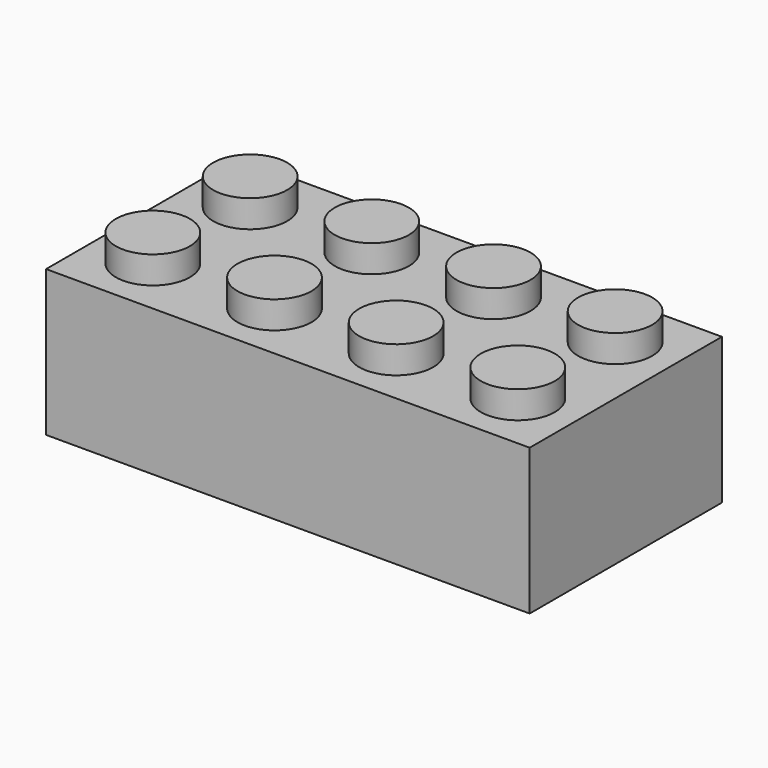
from build123d import *

# Parameters (mm, degrees)
F0_W        = 31.8
F0_H        = 15.8
F1_DEPTH    = 9.6
F2_R        = 2.435
F3_DEPTH    = 1.8
F4_T        = -1.24
F5_R        = 3.2
F6_DEPTH    = 8.36
F7_T        = 1.24
F7_T3_DEPTH = 10.84
F7_T5_DEPTH = 15.8
F7_T7_DEPTH = 31.8


# Not quite as in the source:
# - a shell that OpenCascade refuses in one call is made with other operations: the cavity is built on its own and cut out


with BuildPart() as f1:
    # F0 (on Top) → F1 (new body)
    with BuildSketch(Plane.XY):
        with Locations((15.9, 7.9)):
            Rectangle(F0_W, F0_H)
    extrude(amount=F1_DEPTH)

    # F2 (on face) → F3 (join)
    with BuildSketch(Plane.XY.offset(9.6)):
        with Locations((3.9, 11.9)):
            Circle(F2_R)
        with Locations((11.9, 11.9)):
            Circle(F2_R)
        with Locations((19.9, 11.9)):
            Circle(F2_R)
        with Locations((27.9, 11.9)):
            Circle(F2_R)
        with Locations((27.9, 3.9)):
            Circle(F2_R)
        with Locations((19.9, 3.9)):
            Circle(F2_R)
        with Locations((11.9, 3.9)):
            Circle(F2_R)
        with Locations((3.9, 3.9)):
            Circle(F2_R)
    extrude(amount=F3_DEPTH)

    # F4
    f4_openings = [f1.faces().sort_by_distance(p)[0] for p in [
        (15.9, 7.9, 0),
    ]]
    offset(amount=F4_T, openings=f4_openings, kind=Kind.INTERSECTION)

    # F5 (on face) → F6 (join)
    with BuildSketch(Plane(origin=(0, 0, 8.36), x_dir=(1, 0, 0), z_dir=(0, 0, -1))):
        with Locations((7.9, -7.9)):
            Circle(F5_R)
        with Locations((15.9, -7.9)):
            Circle(F5_R)
        with Locations((23.9, -7.9)):
            Circle(F5_R)
    extrude(amount=F6_DEPTH)

    # F7: shell of thickness 1.24, made by hand


with BuildPart() as f7_core1:
    # F7_t2: copy of F1
    add(f1.part)

    # the walls: a layer under each face that stays
    f7_faces = [f7_core1.faces().sort_by_distance(p)[0] for p in [
        (0, 7.9, 4.8),
        (15.9, 15.8, 4.8),
        (15.9, 0, 4.8),
        (2.2714285714, 1.1285714286, 0),
        (15.9, 7.9, 9.6),
        (31.8, 7.9, 4.8),
        (1.24, 7.9, 4.18),
        (15.9, 14.56, 4.18),
        (30.56, 7.9, 4.18),
        (15.9, 1.24, 4.18),
        (1.465, 3.9, 10.5),
        (9.465, 3.9, 10.5),
        (17.465, 3.9, 10.5),
        (25.465, 3.9, 10.5),
        (1.465, 11.9, 10.5),
        (9.465, 11.9, 10.5),
        (17.465, 11.9, 10.5),
        (25.465, 11.9, 10.5),
        (6.1266666667, 3.46, 8.36),
        (3.9, 3.9, 11.4),
        (11.9, 3.9, 11.4),
        (19.9, 3.9, 11.4),
        (27.9, 3.9, 11.4),
        (3.9, 11.9, 11.4),
        (11.9, 11.9, 11.4),
        (19.9, 11.9, 11.4),
        (27.9, 11.9, 11.4),
        (2.705, 3.9, 9.26),
        (10.705, 3.9, 9.26),
        (18.705, 3.9, 9.26),
        (26.705, 3.9, 9.26),
        (4.7, 7.9, 4.18),
        (2.705, 11.9, 9.26),
        (10.705, 11.9, 9.26),
        (12.7, 7.9, 4.18),
        (20.7, 7.9, 4.18),
        (18.705, 11.9, 9.26),
        (26.705, 11.9, 9.26),
        (3.9, 3.9, 10.16),
        (11.9, 3.9, 10.16),
        (19.9, 3.9, 10.16),
        (27.9, 3.9, 10.16),
        (3.9, 11.9, 10.16),
        (11.9, 11.9, 10.16),
        (19.9, 11.9, 10.16),
        (27.9, 11.9, 10.16),
    ]]
    thicken(f7_faces, amount=-F7_T, mode=Mode.SUBTRACT)

    # F7_s4 → F7_t3 (cut)
    with BuildSketch(Plane.XY.offset(-1.24)):
        Polygon((1.2524, 14.5476), (0, 14.56), (0, 15.8), (1.24, 15.8), align=None)
        Polygon((1.2524, 1.2524), (0, 1.24), (0, 0), (1.24, 0), align=None)
        Polygon((30.5476, 14.5476), (30.56, 15.8), (31.8, 15.8), (31.8, 14.56), align=None)
        Polygon((30.5476, 1.2524), (31.8, 1.24), (31.8, 0), (30.56, 0), align=None)
    extrude(amount=F7_T3_DEPTH, mode=Mode.SUBTRACT)

    # F7_s6 → F7_t5 (cut)
    with BuildSketch(Plane.XZ.offset(-15.8)):
        Polygon((1.2524, 8.3476), (0, 8.36), (0, 9.6), (1.24, 9.6), align=None)
        Polygon((30.5476, 8.3476), (31.8, 8.36), (31.8, 9.6), (30.56, 9.6), align=None)
    extrude(amount=F7_T5_DEPTH, mode=Mode.SUBTRACT)

    # F7_s8 → F7_t7 (cut)
    with BuildSketch(Plane.YZ):
        Polygon((14.5476, 8.3476), (15.8, 8.36), (15.8, 9.6), (14.56, 9.6), align=None)
        Polygon((1.2524, 8.3476), (0, 8.36), (0, 9.6), (1.24, 9.6), align=None)
    extrude(amount=F7_T7_DEPTH, mode=Mode.SUBTRACT)

    # F7_s9 → F7_t10 (revolve, cut)
    with BuildSketch(Plane.XZ.offset(-3.9)):
        Polygon((6.3474, 9.6124), (6.335, 8.36), (5.095, 8.36), (5.095, 9.6), align=None)
    revolve(axis=Axis((3.9, 3.9, 9.6), (0, 0, 1)), mode=Mode.SUBTRACT)

    # F7_s11 → F7_t12 (revolve, cut)
    with BuildSketch(Plane.XZ.offset(-3.9)):
        Polygon((14.3474, 9.6124), (14.335, 8.36), (13.095, 8.36), (13.095, 9.6), align=None)
    revolve(axis=Axis((11.9, 3.9, 9.6), (0, 0, 1)), mode=Mode.SUBTRACT)

    # F7_s13 → F7_t14 (revolve, cut)
    with BuildSketch(Plane.XZ.offset(-3.9)):
        Polygon((22.3474, 9.6124), (22.335, 8.36), (21.095, 8.36), (21.095, 9.6), align=None)
    revolve(axis=Axis((19.9, 3.9, 9.6), (0, 0, 1)), mode=Mode.SUBTRACT)

    # F7_s15 → F7_t16 (revolve, cut)
    with BuildSketch(Plane.XZ.offset(-3.9)):
        Polygon((30.3474, 9.6124), (30.335, 8.36), (29.095, 8.36), (29.095, 9.6), align=None)
    revolve(axis=Axis((27.9, 3.9, 9.6), (0, 0, 1)), mode=Mode.SUBTRACT)

    # F7_s17 → F7_t18 (revolve, cut)
    with BuildSketch(Plane.XZ.offset(-11.9)):
        Polygon((6.3474, 9.6124), (6.335, 8.36), (5.095, 8.36), (5.095, 9.6), align=None)
    revolve(axis=Axis((3.9, 11.9, 9.6), (0, 0, 1)), mode=Mode.SUBTRACT)

    # F7_s19 → F7_t20 (revolve, cut)
    with BuildSketch(Plane.XZ.offset(-11.9)):
        Polygon((14.3474, 9.6124), (14.335, 8.36), (13.095, 8.36), (13.095, 9.6), align=None)
    revolve(axis=Axis((11.9, 11.9, 9.6), (0, 0, 1)), mode=Mode.SUBTRACT)

    # F7_s21 → F7_t22 (revolve, cut)
    with BuildSketch(Plane.XZ.offset(-11.9)):
        Polygon((22.3474, 9.6124), (22.335, 8.36), (21.095, 8.36), (21.095, 9.6), align=None)
    revolve(axis=Axis((19.9, 11.9, 9.6), (0, 0, 1)), mode=Mode.SUBTRACT)

    # F7_s23 → F7_t24 (revolve, cut)
    with BuildSketch(Plane.XZ.offset(-11.9)):
        Polygon((30.3474, 9.6124), (30.335, 8.36), (29.095, 8.36), (29.095, 9.6), align=None)
    revolve(axis=Axis((27.9, 11.9, 9.6), (0, 0, 1)), mode=Mode.SUBTRACT)

    # F7_s25 → F7_t26 (revolve, cut)
    with BuildSketch(Plane.XZ.offset(-7.9)):
        Polygon((11.1124, 8.3476), (11.1, 9.6), (9.86, 9.6), (9.86, 8.36), align=None)
    revolve(axis=Axis((7.9, 7.9, 8.36), (0, 0, -1)), mode=Mode.SUBTRACT)

    # F7_s27 → F7_t28 (revolve, cut)
    with BuildSketch(Plane.XZ.offset(-7.9)):
        Polygon((19.1124, 8.3476), (19.1, 9.6), (17.86, 9.6), (17.86, 8.36), align=None)
    revolve(axis=Axis((15.9, 7.9, 8.36), (0, 0, -1)), mode=Mode.SUBTRACT)

    # F7_s29 → F7_t30 (revolve, cut)
    with BuildSketch(Plane.XZ.offset(-7.9)):
        Polygon((27.1124, 8.3476), (27.1, 9.6), (25.86, 9.6), (25.86, 8.36), align=None)
    revolve(axis=Axis((23.9, 7.9, 8.36), (0, 0, -1)), mode=Mode.SUBTRACT)

    # F7_s31 → F7_t32 (revolve, cut)
    with BuildSketch(Plane.XZ.offset(-3.9)):
        Polygon((5.0826, 10.1476), (6.335, 10.16), (6.335, 11.4), (5.095, 11.4), align=None)
    revolve(axis=Axis((3.9, 3.9, 10.16), (0, 0, -1)), mode=Mode.SUBTRACT)

    # F7_s33 → F7_t34 (revolve, cut)
    with BuildSketch(Plane.XZ.offset(-3.9)):
        Polygon((13.0826, 10.1476), (14.335, 10.16), (14.335, 11.4), (13.095, 11.4), align=None)
    revolve(axis=Axis((11.9, 3.9, 10.16), (0, 0, -1)), mode=Mode.SUBTRACT)

    # F7_s35 → F7_t36 (revolve, cut)
    with BuildSketch(Plane.XZ.offset(-3.9)):
        Polygon((21.0826, 10.1476), (22.335, 10.16), (22.335, 11.4), (21.095, 11.4), align=None)
    revolve(axis=Axis((19.9, 3.9, 10.16), (0, 0, -1)), mode=Mode.SUBTRACT)

    # F7_s37 → F7_t38 (revolve, cut)
    with BuildSketch(Plane.XZ.offset(-3.9)):
        Polygon((29.0826, 10.1476), (30.335, 10.16), (30.335, 11.4), (29.095, 11.4), align=None)
    revolve(axis=Axis((27.9, 3.9, 10.16), (0, 0, -1)), mode=Mode.SUBTRACT)

    # F7_s39 → F7_t40 (revolve, cut)
    with BuildSketch(Plane.XZ.offset(-11.9)):
        Polygon((5.0826, 10.1476), (6.335, 10.16), (6.335, 11.4), (5.095, 11.4), align=None)
    revolve(axis=Axis((3.9, 11.9, 10.16), (0, 0, -1)), mode=Mode.SUBTRACT)

    # F7_s41 → F7_t42 (revolve, cut)
    with BuildSketch(Plane.XZ.offset(-11.9)):
        Polygon((13.0826, 10.1476), (14.335, 10.16), (14.335, 11.4), (13.095, 11.4), align=None)
    revolve(axis=Axis((11.9, 11.9, 10.16), (0, 0, -1)), mode=Mode.SUBTRACT)

    # F7_s43 → F7_t44 (revolve, cut)
    with BuildSketch(Plane.XZ.offset(-11.9)):
        Polygon((21.0826, 10.1476), (22.335, 10.16), (22.335, 11.4), (21.095, 11.4), align=None)
    revolve(axis=Axis((19.9, 11.9, 10.16), (0, 0, -1)), mode=Mode.SUBTRACT)

    # F7_s45 → F7_t46 (revolve, cut)
    with BuildSketch(Plane.XZ.offset(-11.9)):
        Polygon((29.0826, 10.1476), (30.335, 10.16), (30.335, 11.4), (29.095, 11.4), align=None)
    revolve(axis=Axis((27.9, 11.9, 10.16), (0, 0, -1)), mode=Mode.SUBTRACT)


with BuildPart() as f1_1:
    add(f1.part)

    # what is left inside the walls is the cavity
    f7_cavity = [f7_core1.part.solids().sort_by_distance(p)[0] for p in [
        (5.9524, 7.9, 2.786667),
        (13.9524, 7.9, 2.786667),
        (21.9524, 7.9, 2.786667),
    ]]
    add(f7_cavity, mode=Mode.SUBTRACT)


solid = f1_1.part
